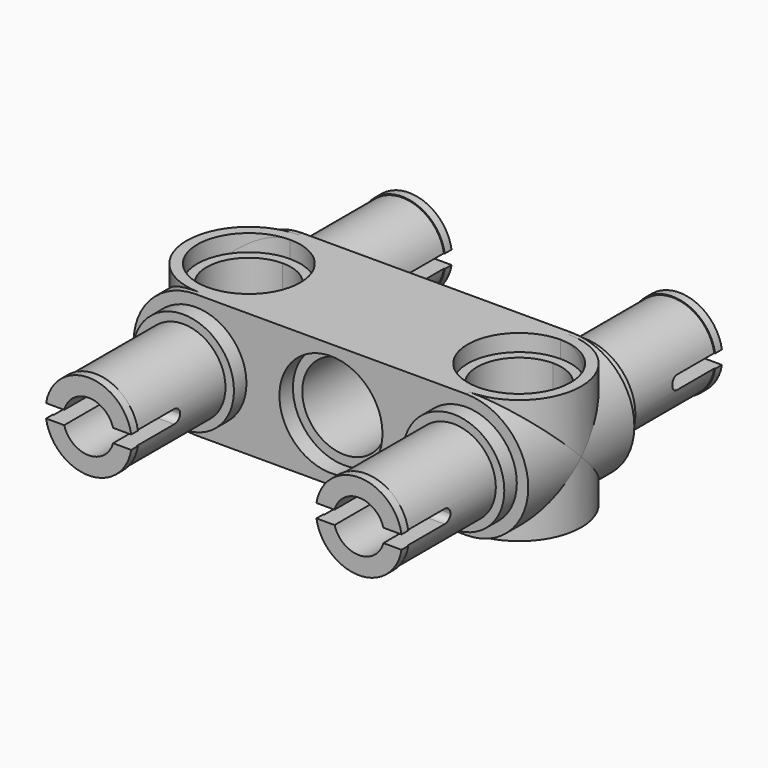
from build123d import *

# Parameters (mm, degrees)
F0_R      = 3.05
F0_R_2    = 3
F0_R_3    = 2.499
F1_DEPTH  = 3.925
F2_DEPTH  = 4.85
F3_DEPTH  = 11.25
F4_R      = 2.55
F5_DEPTH  = 0.6
F6_R      = 2.55
F7_DEPTH  = 0.6
F8_R      = 2.55
F9_DEPTH  = 0.6
F10_R     = 2.55
F11_DEPTH = 0.6
F12_R     = 1.5
F13_DEPTH = 7.925
F14_R     = 1.5
F15_DEPTH = 7.925
F16_R     = 1.5
F17_DEPTH = 7.925
F18_R     = 1.5
F19_DEPTH = 7.925
F20_R     = 3.675
F20_R_2   = 3.05
F21_DEPTH = 7.35
F22_DEPTH = 7.3510001
F23_DEPTH = 1
F25_DEPTH = 1
F26_R     = 3.05
F26_R_2   = 2.499
F27_DEPTH = 1
F28_R     = 3.05
F28_R_2   = 2.499
F29_DEPTH = 1
F30_R     = 2.499
F31_DEPTH = 5.35
F32_R     = 2.499
F33_DEPTH = 5.35
F34_W     = 3.65
F34_H     = 0.8
F35_DEPTH = 12.5
F36_R     = 0.3999
F37_DEPTH = 0.1
F38_DEPTH = 0.1


# Not quite as in the source:
# - a fillet or chamfer is up to 0.001 mm smaller than in the source, because OpenCascade refuses the exact size


with BuildPart() as f1:
    # F0 (on Front) → F1 (new body, symmetric)
    with BuildSketch(Plane.XZ):
        with BuildLine():
            ThreePointArc((8, -3.675), (4.325, 0), (8, 3.675))
            Line((8, 3.675), (-8.0000000262, 3.675))
            ThreePointArc((-8.0000000262, 3.675), (-5.4013825884, 2.5986174301), (-4.325, 0))
            ThreePointArc((-4.325, 0), (-5.4013825791, -2.5986174209), (-8, -3.675))
            Line((-8, -3.675), (8, -3.675))
        make_face()
        Circle(F0_R, mode=Mode.SUBTRACT)
        with BuildLine():
            ThreePointArc((-4.325, 0), (-5.4013825884, 2.5986174301), (-8.0000000262, 3.675))
            ThreePointArc((-8.0000000262, 3.675), (-10.5986174301, 2.5986174116), (-11.675, 0))
            ThreePointArc((-11.675, 0), (-10.5986174209, -2.5986174209), (-8, -3.675))
            ThreePointArc((-8, -3.675), (-5.4013825791, -2.5986174209), (-4.325, 0))
        make_face()
        with Locations((-8, 0)):
            Circle(F0_R_2, mode=Mode.SUBTRACT)
        with BuildLine():
            ThreePointArc((11.675, 0), (10.5986174209, 2.5986174209), (8, 3.675))
            ThreePointArc((8, 3.675), (4.325, 0), (8, -3.675))
            ThreePointArc((8, -3.675), (10.5986174209, -2.5986174209), (11.675, 0))
        make_face()
        with Locations((8, 0)):
            Circle(F0_R_2, mode=Mode.SUBTRACT)
        Circle(F0_R)
        Circle(F0_R_3, mode=Mode.SUBTRACT)
    extrude(amount=F1_DEPTH, both=True)

    # F0 (on Front) → F2 (join, symmetric)
    with BuildSketch(Plane.XZ):
        with Locations((-8, 0)):
            Circle(F0_R_2)
        with Locations((-8, 0)):
            Circle(F0_R_3, mode=Mode.SUBTRACT)
        with Locations((8, 0)):
            Circle(F0_R_2)
        with Locations((8, 0)):
            Circle(F0_R_3, mode=Mode.SUBTRACT)
    extrude(amount=F2_DEPTH, both=True)

    # F0 (on Front) → F3 (join, symmetric)
    with BuildSketch(Plane.XZ):
        with Locations((-8, 0)):
            Circle(F0_R_3)
        with Locations((8, 0)):
            Circle(F0_R_3)
    extrude(amount=F3_DEPTH, both=True)

    # F4 (on face) → F5 (join)
    with BuildSketch(Plane.XZ.offset(11.25)):
        with Locations((-8, 0)):
            Circle(F4_R)
    extrude(amount=F5_DEPTH)

    # F6 (on face) → F7 (join)
    with BuildSketch(Plane.XZ.offset(11.25)):
        with Locations((8, 0)):
            Circle(F6_R)
    extrude(amount=F7_DEPTH)

    # F8 (on face) → F9 (join)
    with BuildSketch(Plane(origin=(0, 11.25, 0), x_dir=(-1, 0, 0), z_dir=(0, 1, 0))):
        with Locations((8, 0)):
            Circle(F8_R)
    extrude(amount=F9_DEPTH)

    # F10 (on face) → F11 (join)
    with BuildSketch(Plane(origin=(0, 11.25, 0), x_dir=(-1, 0, 0), z_dir=(0, 1, 0))):
        with Locations((-8, 0)):
            Circle(F10_R)
    extrude(amount=F11_DEPTH)

    # F12 (on face) → F13 (cut, through all)
    with BuildSketch(Plane(origin=(0, 11.85, 0), x_dir=(-1, 0, 0), z_dir=(0, 1, 0))):
        with Locations((8, 0)):
            Circle(F12_R)
    extrude(amount=-F13_DEPTH, mode=Mode.SUBTRACT)

    # F14 (on face) → F15 (cut, through all)
    with BuildSketch(Plane(origin=(0, 11.85, 0), x_dir=(-1, 0, 0), z_dir=(0, 1, 0))):
        with Locations((-8, 0)):
            Circle(F14_R)
    extrude(amount=-F15_DEPTH, mode=Mode.SUBTRACT)

    # F16 (on face) → F17 (cut, through all)
    with BuildSketch(Plane.XZ.offset(11.85)):
        with Locations((8, 0)):
            Circle(F16_R)
    extrude(amount=-F17_DEPTH, mode=Mode.SUBTRACT)

    # F18 (on face) → F19 (cut, through all)
    with BuildSketch(Plane.XZ.offset(11.85)):
        with Locations((-8, 0)):
            Circle(F18_R)
    extrude(amount=-F19_DEPTH, mode=Mode.SUBTRACT)

    # F20 (on face) → F21 (join, through all)
    with BuildSketch(Plane.XY.offset(3.675)):
        with Locations((-8, 0)):
            Circle(F20_R)
        with Locations((-8, 0)):
            Circle(F20_R_2, mode=Mode.SUBTRACT)
        with Locations((8, 0)):
            Circle(F20_R)
        with Locations((8, 0)):
            Circle(F20_R_2, mode=Mode.SUBTRACT)
    extrude(amount=-F21_DEPTH)

    # F20 (on face) → F22 (cut, through all)
    with BuildSketch(Plane.XY.offset(3.675)):
        with BuildLine():
            Line((-8.0000000262, -2.499), (-8.0000000262, 2.499))
            ThreePointArc((-8.0000000262, 2.499), (-10.499, 0), (-8.0000000262, -2.499))
        make_face()
        with BuildLine():
            ThreePointArc((-5.501, 0), (-6.2329401631, 1.7670598554), (-8.0000000262, 2.499))
            Line((-8.0000000262, 2.499), (-8.0000000262, -2.499))
            ThreePointArc((-8.0000000262, -2.499), (-6.2329401631, -1.7670598554), (-5.501, 0))
        make_face()
        with BuildLine():
            ThreePointArc((10.499, 0), (9.7670598462, 1.7670598462), (8, 2.499))
            Line((8, 2.499), (8, -2.499))
            ThreePointArc((8, -2.499), (9.7670598462, -1.7670598462), (10.499, 0))
        make_face()
        with BuildLine():
            Line((8, -2.499), (8, 2.499))
            ThreePointArc((8, 2.499), (5.501, 0), (8, -2.499))
        make_face()
    extrude(amount=-F22_DEPTH, mode=Mode.SUBTRACT)

    # F20 (on face) → F23 (cut)
    with BuildSketch(Plane.XY.offset(3.675)):
        with BuildLine():
            ThreePointArc((-4.95, 0), (-5.8433243266, 2.1566756919), (-8.0000000262, 3.05))
            Line((-8.0000000262, 3.05), (-8.0000000262, 2.499))
            ThreePointArc((-8.0000000262, 2.499), (-6.2329401631, 1.7670598554), (-5.501, 0))
            ThreePointArc((-5.501, 0), (-6.2329401631, -1.7670598554), (-8.0000000262, -2.499))
            Line((-8.0000000262, -2.499), (-8.0000000262, -3.05))
            ThreePointArc((-8.0000000262, -3.05), (-5.8433243266, -2.1566756919), (-4.95, 0))
        make_face()
        with BuildLine():
            ThreePointArc((11.05, 0), (10.1566756826, 2.1566756826), (8, 3.05))
            Line((8, 3.05), (8, 2.499))
            ThreePointArc((8, 2.499), (9.7670598462, 1.7670598462), (10.499, 0))
            ThreePointArc((10.499, 0), (9.7670598462, -1.7670598462), (8, -2.499))
            Line((8, -2.499), (8, -3.05))
            ThreePointArc((8, -3.05), (10.1566756826, -2.1566756826), (11.05, 0))
        make_face()
        with BuildLine():
            Line((8, 2.499), (8, 3.05))
            ThreePointArc((8, 3.05), (4.95, 0), (8, -3.05))
            Line((8, -3.05), (8, -2.499))
            ThreePointArc((8, -2.499), (5.501, 0), (8, 2.499))
        make_face()
        with BuildLine():
            Line((-8.0000000262, 2.499), (-8.0000000262, 3.05))
            ThreePointArc((-8.0000000262, 3.05), (-11.05, 0), (-8.0000000262, -3.05))
            Line((-8.0000000262, -3.05), (-8.0000000262, -2.499))
            ThreePointArc((-8.0000000262, -2.499), (-10.499, 0), (-8.0000000262, 2.499))
        make_face()
    extrude(amount=-F23_DEPTH, mode=Mode.SUBTRACT)

    # F24 (on face) → F25 (cut)
    with BuildSketch(Plane(origin=(0, 0, -3.675), x_dir=(1, 0, 0), z_dir=(0, 0, -1))):
        with BuildLine():
            ThreePointArc((-8, -3.05), (-5.8433243174, -2.1566756826), (-4.95, 0))
            ThreePointArc((-4.95, 0), (-5.8433243174, 2.1566756826), (-8, 3.05))
            Line((-8, 3.05), (-8, 2.499))
            ThreePointArc((-8.0000000131, 2.499), (-6.2329401584, 1.7670598508), (-5.501, 0))
            ThreePointArc((-5.501, 0), (-6.2329401538, -1.7670598462), (-8, -2.499))
            Line((-8, -2.499), (-8, -3.05))
        make_face()
        with BuildLine():
            Line((-8, 2.499), (-8, 3.05))
            ThreePointArc((-8, 3.05), (-11.05, 0), (-8, -3.05))
            Line((-8, -3.05), (-8, -2.499))
            ThreePointArc((-8, -2.499), (-10.499, -6.5e-09), (-8.0000000131, 2.499))
        make_face()
        with BuildLine():
            ThreePointArc((8, 2.499), (9.7670598462, 1.7670598462), (10.499, 0))
            ThreePointArc((10.499, 0), (9.7670598462, -1.7670598462), (8, -2.499))
            Line((8, -2.499), (8, -3.05))
            ThreePointArc((8, -3.05), (10.1566756826, -2.1566756826), (11.05, 0))
            ThreePointArc((11.05, 0), (10.1566756826, 2.1566756826), (8, 3.05))
            Line((8, 3.05), (8, 2.499))
        make_face()
        with BuildLine():
            ThreePointArc((8, -2.499), (5.501, 0), (8, 2.499))
            Line((8, 2.499), (8, 3.05))
            ThreePointArc((8, 3.05), (4.95, 0), (8, -3.05))
            Line((8, -3.05), (8, -2.499))
        make_face()
    extrude(amount=-F25_DEPTH, mode=Mode.SUBTRACT)

    # F26 (on face) → F27 (cut)
    with BuildSketch(Plane(origin=(0, 3.925, 0), x_dir=(-1, 0, 0), z_dir=(0, 1, 0))):
        Circle(F26_R)
        Circle(F26_R_2, mode=Mode.SUBTRACT)
    extrude(amount=-F27_DEPTH, mode=Mode.SUBTRACT)

    # F28 (on face) → F29 (cut)
    with BuildSketch(Plane.XZ.offset(3.925)):
        Circle(F28_R)
        Circle(F28_R_2, mode=Mode.SUBTRACT)
    extrude(amount=-F29_DEPTH, mode=Mode.SUBTRACT)

    # F30 (on face) → F31 (join, through all)
    with BuildSketch(Plane.XY.offset(2.675)):
        with BuildLine():
            Line((10.5199206337, -1.7182840272), (10.5199206337, 1.7182840275))
            ThreePointArc((10.5199206338, 1.7182840275), (4.95, -1e-10), (10.519920634, -1.7182840272))
        make_face()
        with Locations((8, 0)):
            Circle(F30_R, mode=Mode.SUBTRACT)
        with BuildLine():
            ThreePointArc((10.519920634, -1.7182840272), (10.9144688996, -0.899094563), (11.05, 0))
            ThreePointArc((11.05, 0), (10.9144688996, 0.8990945631), (10.5199206338, 1.7182840275))
            Line((10.5199206337, 1.7182840275), (10.5199206337, -1.7182840272))
        make_face()
    extrude(amount=-F31_DEPTH)

    # F32 (on face) → F33 (join, through all)
    with BuildSketch(Plane.XY.offset(2.675)):
        with BuildLine():
            ThreePointArc((-10.5199206338, -1.7182840275), (-7.1009054369, -2.9144688996), (-4.95, 0))
            ThreePointArc((-4.95, 0), (-7.100905437, 2.9144688996), (-10.519920634, 1.7182840273))
            Line((-10.5199206337, 1.7182840272), (-10.5199206337, -1.7182840275))
        make_face()
        with Locations((-8, 0)):
            Circle(F32_R, mode=Mode.SUBTRACT)
        with BuildLine():
            Line((-10.5199206337, -1.7182840275), (-10.5199206337, 1.7182840272))
            ThreePointArc((-10.519920634, 1.7182840273), (-11.05, -1e-10), (-10.5199206338, -1.7182840275))
        make_face()
    extrude(amount=-F33_DEPTH)

    # F34 (on Right) → F35 (cut, symmetric)
    with BuildSketch(Plane.YZ):
        with Locations((10.025, 0)):
            Rectangle(F34_W, F34_H)
        with Locations((-10.025, 0)):
            Rectangle(F34_W, F34_H)
    extrude(amount=F35_DEPTH, both=True, mode=Mode.SUBTRACT)

    # F36 (radius 0.4 in the source; OpenCascade refuses exactly that, so slightly less here)
    f36_edges = [f1.edges().sort_by_distance(p)[0] for p in [
        (9.956231, 8.2, -0.4),
        (6.043769, 8.2, -0.4),
        (9.956231, 8.2, 0.4),
        (6.043769, 8.2, 0.4),
        (-6.043769, 8.2, 0.4),
        (-9.956231, 8.2, 0.4),
        (9.956231, -8.2, 0.4),
        (6.043769, -8.2, 0.4),
        (-6.043769, 8.2, -0.4),
        (-9.956231, 8.2, -0.4),
        (9.956231, -8.2, -0.4),
        (6.043769, -8.2, -0.4),
        (-6.043769, -8.2, -0.4),
        (-9.956231, -8.2, -0.4),
        (-6.043769, -8.2, 0.4),
        (-9.956231, -8.2, 0.4),
    ]]
    fillet(f36_edges, radius=F36_R)

    # F37 (cut): faces of the model
    f37_faces = [f1.faces().sort_by_distance(p)[0] for p in [
        (5.5073942344, 11.25, 0.4547654088),
        (8, 11.25, -2.5445234591),
        (-10.4926057656, 11.25, 0.4547654088),
        (-8, 11.25, -2.5445234591),
    ]]
    extrude(f37_faces, amount=-F37_DEPTH, mode=Mode.SUBTRACT)

    # F38 (cut): faces of the model
    f38_faces = [f1.faces().sort_by_distance(p)[0] for p in [
        (-5.5073942344, -11.25, 0.4547654088),
        (-8, -11.25, -2.5445234591),
        (10.4926057656, -11.25, 0.4547654088),
        (8, -11.25, -2.5445234591),
    ]]
    extrude(f38_faces, amount=-F38_DEPTH, mode=Mode.SUBTRACT)


solid = f1.part
